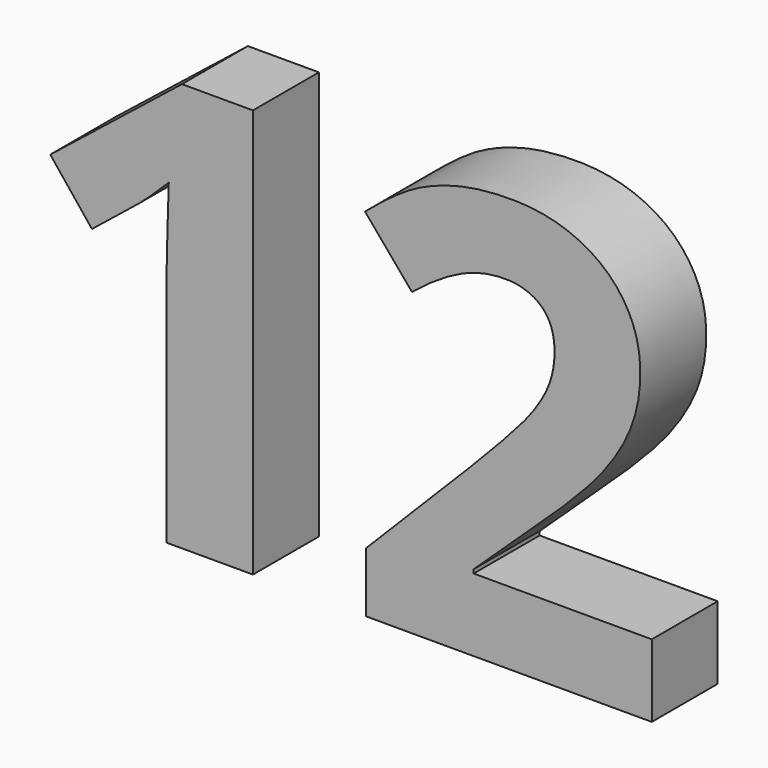
from build123d import *

# Parameters (mm, degrees)
F0_TEXT_SIZE = 35.2777777778
F1_DEPTH     = 5.08


# Not quite as in the source:
# - Text() gives the source's letters only with a copy of the font that has no kerning and outlines rounded to 1/6400 em; it was checked with that copy


with BuildPart() as f1:
    # F0 (on Front) → F1 (new body)
    with BuildSketch(Plane.XZ):
        with Locations((-35.526795798, -13.7237473223)):
            Text('12', F0_TEXT_SIZE, font='Open Sans', font_style=FontStyle.BOLD, text_align=(TextAlign.LEFT, TextAlign.BOTTOM))
    extrude(amount=F1_DEPTH)


solid = f1.part
